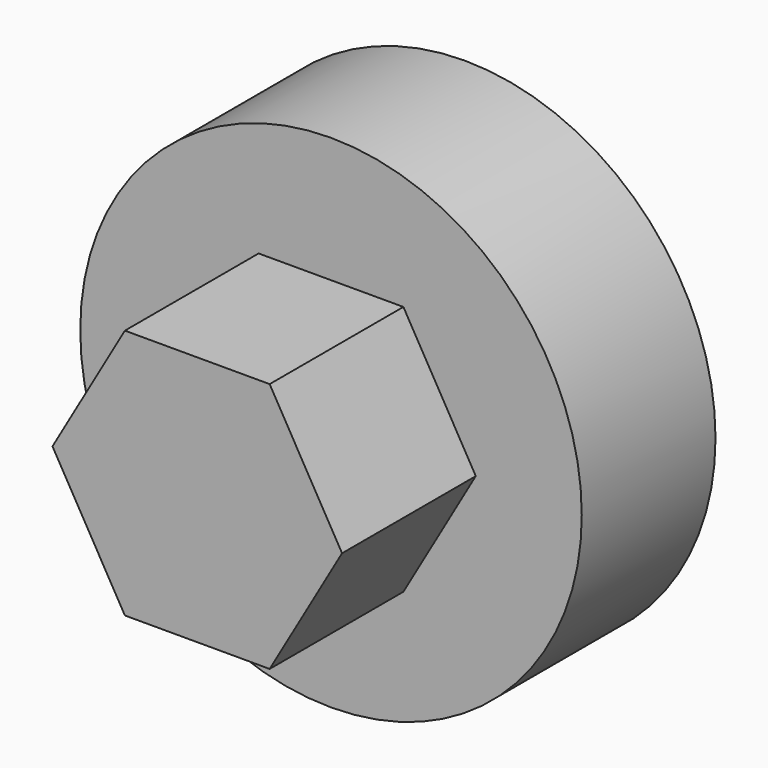
from build123d import *

# Parameters (mm, degrees)
F0_R     = 38.1
F1_DEPTH = 12.7
F3_DEPTH = 25.4


with BuildPart() as f1:
    # F0 (on Front) → F1 (new body, symmetric)
    with BuildSketch(Plane.XZ):
        Circle(F0_R)
    extrude(amount=F1_DEPTH, both=True)

    # F2 (on face) → F3 (join)
    with BuildSketch(Plane.XZ.offset(12.7)):
        Polygon((10.9985226281, 19.05), (-10.9985226281, 19.05), (-21.9970452561, 0), (-10.9985226281, -19.05), (10.9985226281, -19.05), (21.9970452561, 0), align=None)
    extrude(amount=F3_DEPTH)


solid = f1.part
